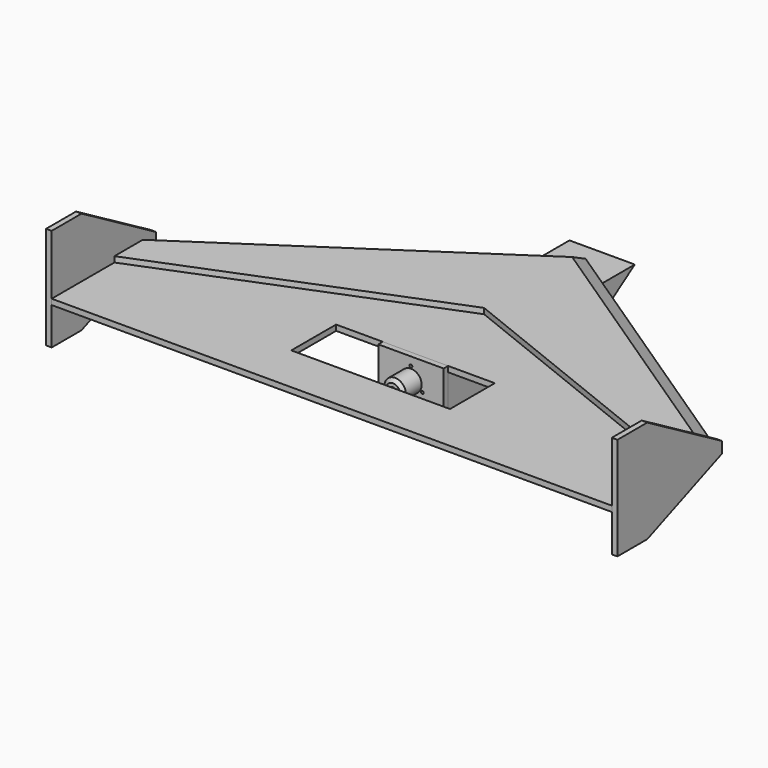
from build123d import *

# Parameters (mm, degrees)
F0_W      = 170
F0_H      = 60
F0_W_2    = 300
F0_H_2    = 40
F1_DEPTH  = 6
F2_DEPTH  = 12
F3_SIZE2  = 9
F3_SIZE   = 15
F4_W      = 70
F4_H      = 250
F5_DEPTH  = 40
F6_SIZE2  = 39.99999
F6_SIZE   = 59.99999
F8_DEPTH  = 6
F10_DEPTH = 6
F11_W     = 70
F11_H     = 40
F11_H_2   = 6
F11_R     = 2.5
F12_DEPTH = 6
F13_R     = 11.5
F13_R_2   = 3.75
F14_DEPTH = 24
F15_SIZE2 = 2.8008301528
F15_SIZE  = 4
F13_R_3   = 2.5
F16_DEPTH = 30
F17_T     = -6


# Not quite as in the source:
# - a fillet or chamfer is up to 0.001 mm smaller than in the source, because OpenCascade refuses the exact size
# - a feature names something its author has since deleted; it is built from what else it names


with BuildPart() as f1:
    # F0 (on Top) → F1 (new body)
    with BuildSketch(Plane.XY):
        Polygon((-300, -86), (-300, -130), (0, -130), (300, -130), (300, -86), (0, 34), align=None)
        with Locations((0, -87.89823)):
            Rectangle(F0_W, F0_H, mode=Mode.SUBTRACT)
        with Locations((-150, -150)):
            Rectangle(F0_W_2, F0_H_2)
        with Locations((150, -150)):
            Rectangle(F0_W_2, F0_H_2)
    extrude(amount=F1_DEPTH)

    # F0 (on Top) → F2 (join)
    with BuildSketch(Plane.XY):
        Polygon((-300, -30), (-300, -86), (0, 34), (300, -86), (300, -30), (0, 170), align=None)
    extrude(amount=F2_DEPTH)

    # F3
    f3_edges = [f1.edges().sort_by_distance(p)[0] for p in [
        (-150, 70, 12),
        (150, 70, 12),
    ]]
    f3_side = f1.faces().sort_by_distance((-293.476688, -58, 12))[0]
    chamfer(f3_edges, length=F3_SIZE, length2=F3_SIZE2, reference=f3_side)


with BuildPart() as f5:
    # F4 (on face) → F5 (new body)
    with BuildSketch(Plane.XY):
        with Locations((0, 67.10177)):
            Rectangle(F4_W, F4_H)
    extrude(amount=-F5_DEPTH)

    # F6 (size 60 and 40 in the source; OpenCascade refuses exactly that, so slightly less here)
    f6_edges = [f5.edges().sort_by_distance(p)[0] for p in [
        (0, 192.10177, -40),
    ]]
    f6_side = f5.faces().sort_by_distance((0, 67.10177, -40))[0]
    chamfer(f6_edges, length=F6_SIZE, length2=F6_SIZE2, reference=f6_side)

    # F17
    f17_openings = [f5.faces().sort_by_distance(p)[0] for p in [
        (0, -57.89823, -20),
    ]]
    offset(amount=F17_T, openings=f17_openings)


with BuildPart() as f8:
    # F7 (on face) → F8 (new body)
    with BuildSketch(Plane.YZ.offset(300)):
        Polygon((-30, 0), (-170, 0), (-170, -40), (-130, -40), align=None)
        Polygon((-130, 70), (-170, 70), (-170, 6), (-86, 6), (-86, 12), (-48.0277563773, 12), (-30, 3), (-30, 12), align=None)
        Polygon((-86, 6), (-170, 6), (-170, 0), (-30, 0), (-30, 3), (-48.0277563773, 12), (-86, 12), align=None)
    extrude(amount=F8_DEPTH)


with BuildPart() as f10:
    # F9 (on face) → F10 (new body)
    with BuildSketch(Plane(origin=(-300, 0, 0), x_dir=(0, -1, 0), z_dir=(-1, 0, 0))):
        Polygon((170, -40), (170, 0), (30, 0), (130, -40), align=None)
        Polygon((86, 6), (170, 6), (170, 70), (130, 70), (30, 12), (30, 3), (48.0277563773, 12), (86, 12), align=None)
        Polygon((30, 0), (170, 0), (170, 6), (86, 6), (86, 12), (48.0277563773, 12), (30, 3), align=None)
    extrude(amount=F10_DEPTH)


with BuildPart() as f12:
    # F11 (on face) → F12 (new body)
    with BuildSketch(Plane.XZ.offset(57.89823)):
        with Locations((0, -20)):
            Rectangle(F11_W, F11_H)
        with BuildLine():
            ThreePointArc((1.49784603, -3.0803571429), (10.4156095458, -7.645050626), (14, -17))
            ThreePointArc((14, -17), (13.6976571495, -19.8938190361), (12.8036873409, -22.6626487156))
            ThreePointArc((12.8036873409, -22.6626487156), (13.4028308252, -23.2154611329), (13.624355653, -24))
            ThreePointArc((13.624355653, -24), (12.8392781966, -25.3186681753), (11.3058413109, -25.2569941415))
            ThreePointArc((11.3058413109, -25.2569941415), (0, -31), (-11.3058413109, -25.2569941415))
            ThreePointArc((-11.3058413109, -25.2569941415), (-13.4233937587, -24.75), (-12.8036873409, -22.6626487156))
            ThreePointArc((-12.8036873409, -22.6626487156), (-12.124355653, -10), (-1.49784603, -3.0803571429))
            ThreePointArc((-1.49784603, -3.0803571429), (-0.0401930031, -1.5005385892), (1.5, -3))
            ThreePointArc((1.5, -3), (1.4994614108, -3.0401930031), (1.49784603, -3.0803571429))
        make_face(mode=Mode.SUBTRACT)
        with Locations((0, 3)):
            Rectangle(F11_W, F11_H_2)
        with BuildLine():
            ThreePointArc((12.8036873409, -22.6626487156), (13.6976571495, -19.8938190361), (14, -17))
            ThreePointArc((14, -17), (10.4156095458, -7.645050626), (1.49784603, -3.0803571429))
            ThreePointArc((1.49784603, -3.0803571429), (0, -4.5), (-1.49784603, -3.0803571429))
            ThreePointArc((-1.49784603, -3.0803571429), (-12.124355653, -10), (-12.8036873409, -22.6626487156))
            ThreePointArc((-12.8036873409, -22.6626487156), (-11.3398167858, -22.7215248278), (-10.624355653, -24))
            ThreePointArc((-10.624355653, -24), (-10.8056874777, -24.7149225437), (-11.3058413109, -25.2569941415))
            ThreePointArc((-11.3058413109, -25.2569941415), (0, -31), (11.3058413109, -25.2569941415))
            ThreePointArc((11.3058413109, -25.2569941415), (10.8253175473, -23.25), (12.8036873409, -22.6626487156))
        make_face()
        with Locations((0, -17)):
            Circle(F11_R, mode=Mode.SUBTRACT)
    extrude(amount=F12_DEPTH)


with BuildPart() as f14:
    # F13 (on face) → F14 (new body)
    with BuildSketch(Plane.XZ.offset(63.89823)):
        with Locations((0, -17.040412873)):
            Circle(F13_R)
        with Locations((0, -17.040412873)):
            Circle(F13_R_2, mode=Mode.SUBTRACT)
    extrude(amount=F14_DEPTH)

    # F15
    f15_edges = [f14.edges().sort_by_distance(p)[0] for p in [
        (-11.5, -87.89823, -17.040413),
    ]]
    f15_side = f14.faces().sort_by_distance((-11.174731, -87.89823, -17.040413))[0]
    chamfer(f15_edges, length=F15_SIZE, length2=F15_SIZE2, reference=f15_side)

    # F13 (on face) → F16 (join)
    with BuildSketch(Plane.XZ.offset(63.89823)):
        with Locations((0, -17.040412873)):
            Circle(F13_R_2)
        with Locations((0, -17)):
            Circle(F13_R_3, mode=Mode.SUBTRACT)
        with Locations((0, -17)):
            Circle(F13_R_3)
    extrude(amount=F16_DEPTH)


solid = Compound([f1.part, f5.part, f8.part, f10.part, f12.part, f14.part])
